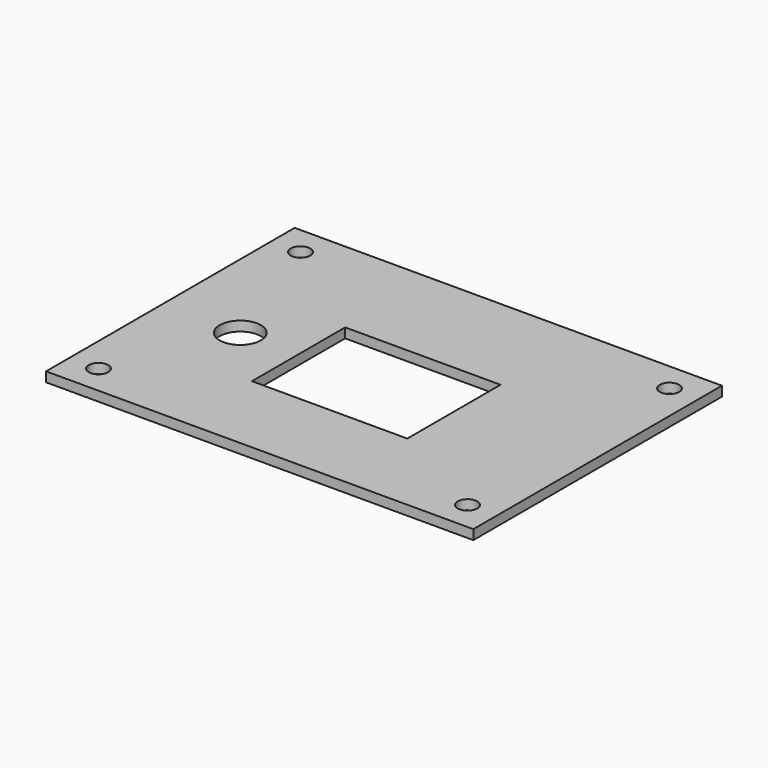
from build123d import *

# Parameters (mm, degrees)
F0_W     = 139.7
F0_H     = 101.6
F0_R     = 3.175
F0_R_2   = 6.746875
F0_W_2   = 50.8
F0_H_2   = 38.1
F1_DEPTH = 3.175


# Not quite as in the source:
# - a feature names something its author has since deleted; it is built from what else it names


with BuildPart() as f1:
    # F0 (on Top) → F1 (new body)
    with BuildSketch(Plane.XY):
        with Locations((69.85, 50.8)):
            Rectangle(F0_W, F0_H)
        with Locations((9.525, 9.525)):
            Circle(F0_R, mode=Mode.SUBTRACT)
        with Locations((25.4, 47.625)):
            Circle(F0_R_2, mode=Mode.SUBTRACT)
        with Locations((130.175, 9.525)):
            Circle(F0_R, mode=Mode.SUBTRACT)
        with Locations((69.85, 47.625)):
            Rectangle(F0_W_2, F0_H_2, mode=Mode.SUBTRACT)
        with Locations((9.525, 92.075)):
            Circle(F0_R, mode=Mode.SUBTRACT)
        with Locations((130.175, 92.075)):
            Circle(F0_R, mode=Mode.SUBTRACT)
    extrude(amount=F1_DEPTH)


solid = f1.part
